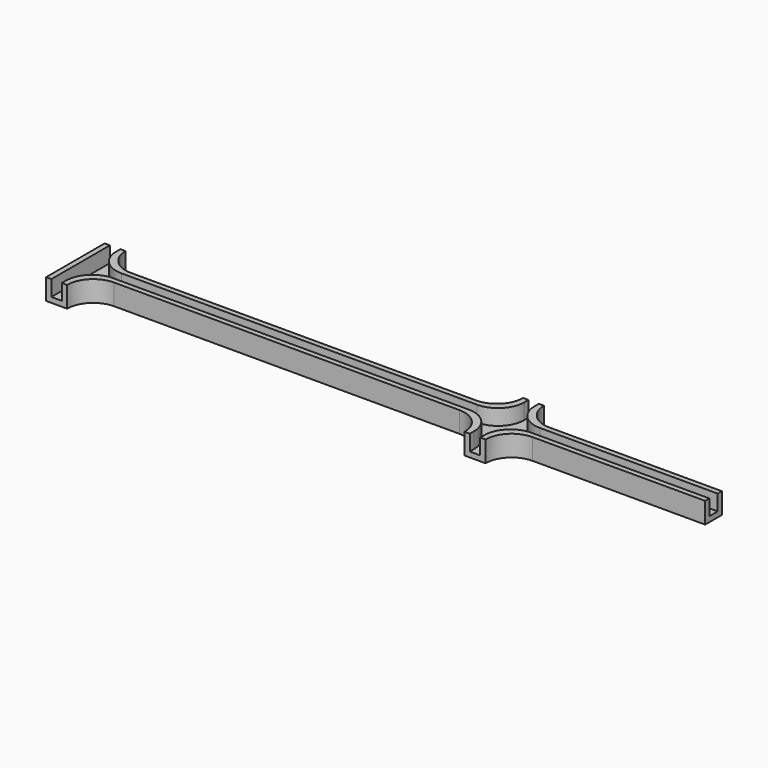
from build123d import *

# Parameters (mm, degrees)
F0_W     = 4
F0_H     = 5
F0_W_2   = 76
F0_H_2   = 2
F1_DEPTH = 1
F2_W     = 1
F2_H     = 14
F2_W_2   = 6
F2_H_2   = 1
F2_W_3   = 5
F2_W_4   = 33
F2_W_5   = 65
F3_DEPTH = 3
F4_R     = 4.99999
F5_R     = 4.99999


# Not quite as in the source:
# - a fillet or chamfer is up to 0.001 mm smaller than in the source, because OpenCascade refuses the exact size


with BuildPart() as f1:
    # F0 (on Top) → F1 (new body)
    with BuildSketch(Plane.XY):
        with Locations((-59, 4.5)):
            Rectangle(F0_W, F0_H)
        with Locations((-19, -1)):
            Rectangle(F0_W_2, F0_H_2)
        with Locations((-19, 1)):
            Rectangle(F0_W_2, F0_H_2)
        with Locations((-59, -1)):
            Rectangle(F0_W, F0_H_2)
        with Locations((-59, 1)):
            Rectangle(F0_W, F0_H_2)
        with Locations((-59, -4.5)):
            Rectangle(F0_W, F0_H)
        Polygon((61, 2), (23, 2), (23, 0), (23, -2), (61, -2), align=None)
        with Locations((21, 1)):
            Rectangle(F0_W, F0_H_2)
        with Locations((21, -1)):
            Rectangle(F0_W, F0_H_2)
        with Locations((21, 4.5)):
            Rectangle(F0_W, F0_H)
        with Locations((21, -4.5)):
            Rectangle(F0_W, F0_H)
    extrude(amount=F1_DEPTH)

    # F2 (on face) → F3 (join)
    with BuildSketch(Plane.XY.offset(1)):
        with Locations((-60.5, 0)):
            Rectangle(F2_W, F2_H)
        Polygon((-57, 7), (-58, 7), (-58, 1), (-57, 1), (-57, 2), align=None)
        with Locations((-54, 1.5)):
            Rectangle(F2_W_2, F2_H_2)
        with Locations((-54, -1.5)):
            Rectangle(F2_W_2, F2_H_2)
        Polygon((-58, -1), (-58, -7), (-57, -7), (-57, -2), (-57, -1), align=None)
        Polygon((19, -1), (19, -2), (19, -7), (20, -7), (20, -1), align=None)
        Polygon((19, 7), (19, 2), (19, 1), (20, 1), (20, 7), align=None)
        with Locations((16.5, 1.5)):
            Rectangle(F2_W_3, F2_H_2)
        with Locations((16.5, -1.5)):
            Rectangle(F2_W_3, F2_H_2)
        with Locations((25.5, -1.5)):
            Rectangle(F2_W_3, F2_H_2)
        with Locations((25.5, 1.5)):
            Rectangle(F2_W_3, F2_H_2)
        Polygon((23, 7), (22, 7), (22, 1), (23, 1), (23, 2), align=None)
        Polygon((22, -1), (22, -7), (23, -7), (23, -2), (23, -1), align=None)
        with Locations((44.5, -1.5)):
            Rectangle(F2_W_4, F2_H_2)
        with Locations((-18.5, 1.5)):
            Rectangle(F2_W_5, F2_H_2)
        with Locations((-18.5, -1.5)):
            Rectangle(F2_W_5, F2_H_2)
        with Locations((44.5, 1.5)):
            Rectangle(F2_W_4, F2_H_2)
    extrude(amount=F3_DEPTH)

    # F4 (radius 5 in the source; OpenCascade refuses exactly that, so slightly less here)
    f4_edges = [f1.edges().sort_by_distance(p)[0] for p in [
        (23, -2, 2),
        (20, -1, 2.5),
        (20, 1, 2.5),
        (22, 1, 2.5),
        (19, -2, 2),
        (22, -1, 2.5),
        (19, 2, 2),
        (23, 2, 2),
    ]]
    fillet(f4_edges, radius=F4_R)

    # F5 (radius 5 in the source; OpenCascade refuses exactly that, so slightly less here)
    f5_edges = [f1.edges().sort_by_distance(p)[0] for p in [
        (-57, -2, 2),
        (-58, 1, 2.5),
        (-57, 2, 2),
        (-58, -1, 2.5),
    ]]
    fillet(f5_edges, radius=F5_R)


solid = f1.part
